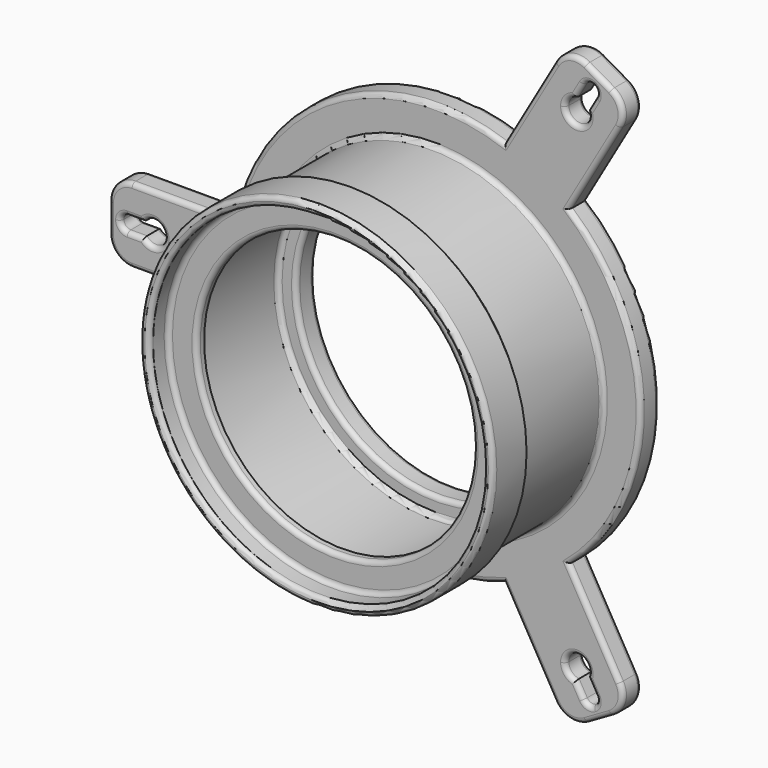
from build123d import *

# Parameters (mm, degrees)
F0_R        = 38
F0_R_2      = 36
F0_R_3      = 31.8
F0_R_4      = 29.8
F1_DEPTH    = 2
F2_DEPTH    = 5
F3_R        = 0.99999
F4_R        = 36
F4_R_2      = 34
F5_DEPTH    = 25
F6_R        = 30
F7_DEPTH    = 5
F8_S7_R     = 38
F8_T8_DEPTH = 58
F9_R        = 1


# Not quite as in the source:
# - a fillet or chamfer that OpenCascade refuses, or shapes differently, is made with other operations: its cross-section is extruded or revolved along the edge and cut away or added
# - a fillet or chamfer is up to 0.001 mm smaller than in the source, because OpenCascade refuses the exact size


with BuildPart() as f1:
    # F0 (on Front) → F1 (new body)
    with BuildSketch(Plane.XZ):
        Circle(F0_R)
        Circle(F0_R_2, mode=Mode.SUBTRACT)
        Circle(F0_R_2)
        Circle(F0_R_3, mode=Mode.SUBTRACT)
        Circle(F0_R_3)
        Circle(F0_R_4, mode=Mode.SUBTRACT)
    extrude(amount=-F1_DEPTH)

    # F0 (on Front) → F2 (join)
    with BuildSketch(Plane.XZ):
        Circle(F0_R)
        Circle(F0_R_2, mode=Mode.SUBTRACT)
    extrude(amount=F2_DEPTH)

    # F3 (radius 1 in the source; OpenCascade refuses exactly that, so slightly less here)
    f3_edges = [f1.edges().sort_by_distance(p)[0] for p in [
        (-38, -5, 0),
        (-36, -5, 0),
        (-36, 0, 0),
        (-29.8, 0, 0),
    ]]
    fillet(f3_edges, radius=F3_R)

    # F4 (on face) → F5 (join)
    with BuildSketch(Plane(origin=(0, 2, 0), x_dir=(-1, 0, 0), z_dir=(0, 1, 0))):
        Circle(F4_R)
        Circle(F4_R_2, mode=Mode.SUBTRACT)
    extrude(amount=F5_DEPTH)

    # F6 (on face) → F7 (join)
    with BuildSketch(Plane(origin=(0, 27, 0), x_dir=(-1, 0, 0), z_dir=(0, 1, 0))):
        with BuildLine():
            ThreePointArc((43.4274953318, -8.0724546886), (43.98502471, -4.0533290955), (44.1713920484, 0))
            ThreePointArc((44.1713920484, 0), (43.98502471, 4.0533290955), (43.4274953318, 8.0724546886))
            Line((43.4274953318, 8.0724546886), (35.0832648894, 8.0724546886))
            Line((35.0832648894, 8.0724546886), (35.0832648894, -8.0724546886))
            Line((35.0832648894, -8.0724546886), (43.4274953318, -8.0724546886))
        make_face()
        with BuildLine():
            ThreePointArc((43.4274953318, 8.0724546886), (43.98502471, 4.0533290955), (44.1713920484, 0))
            ThreePointArc((44.1713920484, 0), (43.98502471, -4.0533290955), (43.4274953318, -8.0724546886))
            Line((43.4274953318, -8.0724546886), (65.2730737311, -8.0724546886))
            ThreePointArc((65.2730737311, -8.0724546886), (68.8086076371, -6.6079885946), (70.2730737311, -3.0724546886))
            Line((70.2730737311, -3.0724546886), (70.2730737311, 3.0724546886))
            ThreePointArc((70.2730737311, 3.0724546886), (68.8086076371, 6.6079885946), (65.2730737311, 8.0724546886))
            Line((65.2730737311, 8.0724546886), (43.4274953318, 8.0724546886))
        make_face()
        with BuildLine():
            ThreePointArc((62.8264366316, -1.5), (58.3264366316, 0), (62.8264366316, 1.5))
            Line((62.8264366316, 1.5), (66.3264366316, 1.5))
            ThreePointArc((66.3264366316, 1.5), (67.3870968033, 1.0606601718), (67.8264366316, 0))
            ThreePointArc((67.8264366316, 0), (67.3870968033, -1.0606601718), (66.3264366316, -1.5))
            Line((66.3264366316, -1.5), (62.8264366316, -1.5))
        make_face(mode=Mode.SUBTRACT)
        with BuildLine():
            Line((35.0832648894, 8.0724546886), (43.4274953318, 8.0724546886))
            ThreePointArc((43.4274953318, 8.0724546886), (22.0856960242, 38.2535476345), (-14.7227968347, 41.6455415244))
            Line((-14.7227968347, 41.6455415244), (-10.5506816135, 34.4192259862))
            Line((-10.5506816135, 34.4192259862), (-24.5325832759, 26.3467712976))
            Line((-24.5325832759, 26.3467712976), (-28.7046984972, 33.5730868358))
            ThreePointArc((-28.7046984972, 33.5730868358), (-44.1713920484, 0), (-28.7046984972, -33.5730868358))
            Line((-28.7046984972, -33.5730868358), (-24.5325832759, -26.3467712976))
            Line((-24.5325832759, -26.3467712976), (-10.5506816135, -34.4192259862))
            Line((-10.5506816135, -34.4192259862), (-14.7227968347, -41.6455415244))
            ThreePointArc((-14.7227968347, -41.6455415244), (22.0856960242, -38.2535476345), (43.4274953318, -8.0724546886))
            Line((43.4274953318, -8.0724546886), (35.0832648894, -8.0724546886))
            Line((35.0832648894, -8.0724546886), (35.0832648894, 8.0724546886))
        make_face()
        Circle(F6_R, mode=Mode.SUBTRACT)
        with BuildLine():
            Line((-10.5506816135, 34.4192259862), (-14.7227968347, 41.6455415244))
            ThreePointArc((-14.7227968347, 41.6455415244), (-22.0856960242, 38.2535476345), (-28.7046984972, 33.5730868358))
            Line((-28.7046984972, 33.5730868358), (-24.5325832759, 26.3467712976))
            Line((-24.5325832759, 26.3467712976), (-10.5506816135, 34.4192259862))
        make_face()
        with BuildLine():
            ThreePointArc((-28.7046984972, 33.5730868358), (-22.0856960242, 38.2535476345), (-14.7227968347, 41.6455415244))
            Line((-14.7227968347, 41.6455415244), (-25.6455860343, 60.5643673786))
            ThreePointArc((-25.6455860343, 60.5643673786), (-28.6816178277, 62.89399651), (-32.4757130532, 62.3944943975))
            Line((-32.4757130532, 62.3944943975), (-37.7973606779, 59.3220397089))
            ThreePointArc((-37.7973606779, 59.3220397089), (-40.1269898093, 56.2860079155), (-39.6274876968, 52.4919126899))
            Line((-39.6274876968, 52.4919126899), (-28.7046984972, 33.5730868358))
        make_face()
        with BuildLine():
            ThreePointArc((-30.1141802101, 55.1592901522), (-28.5427109963, 54.3359142277), (-27.9132183158, 52.6772393446))
            ThreePointArc((-27.9132183158, 52.6772393446), (-30.9144192415, 50.2279950465), (-32.7122564215, 53.6592901522))
            Line((-32.7122564215, 53.6592901522), (-34.4622564215, 56.6903790654))
            ThreePointArc((-34.4622564215, 56.6903790654), (-34.6121070552, 57.8286076331), (-33.9132183158, 58.7394171711))
            ThreePointArc((-33.9132183158, 58.7394171711), (-32.7749897481, 58.8892678049), (-31.8641802101, 58.1903790654))
            Line((-31.8641802101, 58.1903790654), (-30.1141802101, 55.1592901522))
        make_face(mode=Mode.SUBTRACT)
        with BuildLine():
            Line((-25.6455860343, -60.5643673786), (-14.7227968347, -41.6455415244))
            ThreePointArc((-14.7227968347, -41.6455415244), (-22.0856960242, -38.2535476345), (-28.7046984972, -33.5730868358))
            Line((-28.7046984972, -33.5730868358), (-39.6274876968, -52.4919126899))
            ThreePointArc((-39.6274876968, -52.4919126899), (-40.1269898093, -56.2860079155), (-37.7973606779, -59.3220397089))
            Line((-37.7973606779, -59.3220397089), (-32.4757130532, -62.3944943975))
            ThreePointArc((-32.4757130532, -62.3944943975), (-28.6816178277, -62.89399651), (-25.6455860343, -60.5643673786))
        make_face()
        with BuildLine():
            ThreePointArc((-32.7122564215, -53.6592901522), (-30.9144192415, -50.2279950465), (-27.9132183158, -52.6772393446))
            ThreePointArc((-27.9132183158, -52.6772393446), (-28.5427109963, -54.3359142277), (-30.1141802101, -55.1592901522))
            Line((-30.1141802101, -55.1592901522), (-31.8641802101, -58.1903790654))
            ThreePointArc((-31.8641802101, -58.1903790654), (-32.7749897481, -58.8892678049), (-33.9132183158, -58.7394171711))
            ThreePointArc((-33.9132183158, -58.7394171711), (-34.6121070552, -57.8286076331), (-34.4622564215, -56.6903790654))
            Line((-34.4622564215, -56.6903790654), (-32.7122564215, -53.6592901522))
        make_face(mode=Mode.SUBTRACT)
        with BuildLine():
            ThreePointArc((-28.7046984972, -33.5730868358), (-22.0856960242, -38.2535476345), (-14.7227968347, -41.6455415244))
            Line((-14.7227968347, -41.6455415244), (-10.5506816135, -34.4192259862))
            Line((-10.5506816135, -34.4192259862), (-24.5325832759, -26.3467712976))
            Line((-24.5325832759, -26.3467712976), (-28.7046984972, -33.5730868358))
        make_face()
    extrude(amount=F7_DEPTH)

    # F8: chamfer of 4 on 2 edges, made by hand

    # F8_s1 → F8_t2 (revolve)
    with BuildSketch(Plane.XY):
        Polygon((-34, 6), (-30, 2), (-34, 2), align=None)
    revolve(axis=Axis((0, 2, 0), (0, 1, 0)))


with BuildPart() as f8_tool4:
    # F8_s5 → F8_t6 (revolve)
    with BuildSketch(Plane.XY):
        Polygon((-36, 6), (-40, 2), (-36, 2), align=None)
    revolve(axis=Axis((0, 2, 0), (0, 1, 0)))

    # F8_s7 → F8_t8 (intersect, symmetric)
    with BuildSketch(Plane.XZ.offset(-4)):
        Circle(F8_S7_R)
    extrude(amount=F8_T8_DEPTH, both=True, mode=Mode.INTERSECT)


with BuildPart() as f1_1:
    add(f1.part)

    # F8_t3: union F8_tool4
    add(f8_tool4.part)

    # F9
    f9_edges = [f1_1.edges().sort_by_distance(p)[0] for p in [
        (-54.350285, 27, -8.072455),
        (-22.085696, 27, -38.253548),
        (-68.808608, 27, -6.607989),
        (20.184191, 27, -51.104954),
        (-70.273074, 27, 0),
        (28.681618, 27, -62.893997),
        (-68.808608, 27, 6.607989),
        (35.136537, 27, -60.858267),
        (-54.350285, 27, 8.072455),
        (40.12699, 27, -56.286008),
        (-22.085696, 27, 38.253548),
        (34.166093, 27, -43.0325),
        (20.184191, 27, 51.104954),
        (44.171392, 27, 0),
        (28.681618, 27, 62.893997),
        (34.166093, 27, 43.0325),
        (35.136537, 27, 60.858267),
        (40.12699, 27, 56.286008),
        (33.587256, 27, -55.174835),
        (33.913218, 27, -58.739417),
        (29.163218, 27, -50.512176),
        (30.98918, 27, -56.674835),
        (36, 27, 0),
        (-67.826437, 27, 0),
        (-64.576437, 27, 1.5),
        (-64.576437, 27, -1.5),
        (-58.326437, 27, 0),
        (30.98918, 27, 56.674835),
        (33.913218, 27, 58.739417),
        (29.163218, 27, 50.512176),
        (33.587256, 27, 55.174835),
        (-54.350285, 32, -8.072455),
        (-68.808608, 32, -6.607989),
        (-70.273074, 32, 0),
        (-68.808608, 32, 6.607989),
        (-54.350285, 32, 8.072455),
        (-22.085696, 32, 38.253548),
        (20.184191, 32, 51.104954),
        (28.681618, 32, 62.893997),
        (35.136537, 32, 60.858267),
        (40.12699, 32, 56.286008),
        (34.166093, 32, 43.0325),
        (44.171392, 32, 0),
        (34.166093, 32, -43.0325),
        (40.12699, 32, -56.286008),
        (35.136537, 32, -60.858267),
        (28.681618, 32, -62.893997),
        (20.184191, 32, -51.104954),
        (-22.085696, 32, -38.253548),
        (-67.826437, 32, 0),
        (-64.576437, 32, -1.5),
        (-58.326437, 32, 0),
        (-64.576437, 32, 1.5),
        (30, 32, 0),
        (30.98918, 32, 56.674835),
        (29.163218, 32, 50.512176),
        (33.587256, 32, 55.174835),
        (33.913218, 32, 58.739417),
        (33.587256, 32, -55.174835),
        (29.163218, 32, -50.512176),
        (30.98918, 32, -56.674835),
        (33.913218, 32, -58.739417),
        (30, 27, 0),
        (34, 27, 0),
    ]]
    fillet(f9_edges, radius=F9_R)


solid = f1_1.part
